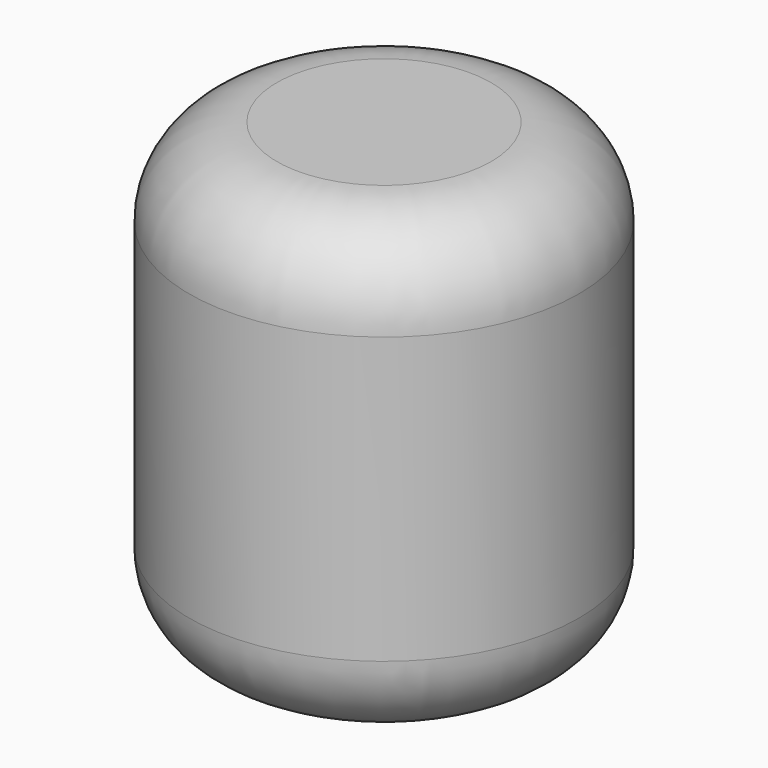
from build123d import *

# Parameters (mm, degrees)
F0_R     = 56.3745675483
F1_DEPTH = 133.35
F2_R     = 25.4
F3_R     = 25.4
F4_T     = -2.54


# Not quite as in the source:
# - a shell that OpenCascade refuses in one call is made with other operations: the cavity is built on its own and cut out


with BuildPart() as f1:
    # F0 (on Top) → F1 (new body)
    with BuildSketch(Plane.XY):
        Circle(F0_R)
    extrude(amount=F1_DEPTH)

    # F2
    f2_edges = [f1.edges().sort_by_distance(p)[0] for p in [
        (-56.374568, 0, 133.35),
    ]]
    fillet(f2_edges, radius=F2_R)

    # F3
    f3_edges = [f1.edges().sort_by_distance(p)[0] for p in [
        (-56.374568, 0, 0),
    ]]
    fillet(f3_edges, radius=F3_R)

    # F4: a shell. OpenCascade refuses it in one call, so the cavity is built on its own and cut out:
    # the body offset inwards by the wall thickness, plus a prism from it out through each open face.
    f4_core = offset(f1.part, amount=F4_T, mode=Mode.PRIVATE)
    f4_exits = [f4_core.faces().sort_by_distance(p)[0] for p in [
        (0, 0, 2.54),
    ]]
    add(f4_core, mode=Mode.SUBTRACT)
    extrude(f4_exits, amount=-F4_T, mode=Mode.SUBTRACT)


solid = f1.part
